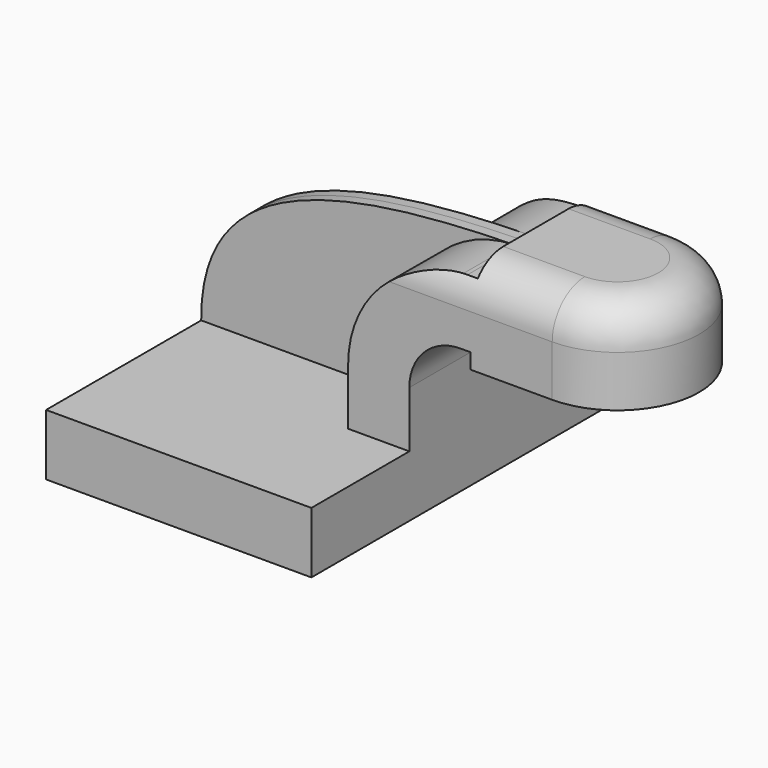
from build123d import *

# Parameters (mm, degrees)
F1_DEPTH = 63.5
F0_W     = 25.4
F0_H     = 19.05
F0_H_2   = 4.7498
F0_H_3   = 4.7752
F2_DEPTH = 25.4
F4_DEPTH = 3.175
F5_R     = 12.7


with BuildPart() as f1:
    # F0 (on Front) → F1 (new body, symmetric)
    with BuildSketch(Plane.XZ):
        Polygon((41.275, -9.525), (41.275, 9.525), (22.225, 9.525), (-41.275, 9.525), (-41.275, -9.525), align=None)
    extrude(amount=F1_DEPTH, both=True)

    # F0 (on Front) → F2 (join, symmetric)
    with BuildSketch(Plane.XZ):
        with BuildLine():
            Line((22.225, 9.525), (41.275, 9.525))
            Line((41.275, 9.525), (41.275, 27.0002))
            ThreePointArc((41.275, 27.0002), (45.9246798487, 38.2255201513), (57.15, 42.8752))
            Line((57.15, 42.8752), (60.325, 42.8752))
            Line((60.325, 42.8752), (60.325, 61.9252))
            Line((60.325, 61.9252), (57.15, 61.9252))
            add(Edge.make_bspline(
                [(55.8906627655, 61.9024878151), (56.3095920905, 61.9105285601), (56.7293746708, 61.9180961221), (57.15, 61.9252)],
                knots=[110.683860184, 110.683860184, 110.683860184, 110.683860184, 111.5045361635, 111.5045361635, 111.5045361635, 111.5045361635], degree=3))
            ThreePointArc((55.8906627655, 61.9024878151), (32.0129956248, 51.2465736679), (22.225, 27.0002))
            Line((22.225, 27.0002), (22.225, 9.525))
        make_face()
        with Locations((73.025, 52.4002)):
            Rectangle(F0_W, F0_H)
        with Locations((73.025, 64.3001)):
            Rectangle(F0_W, F0_H_2)
        with Locations((73.025, 40.4876)):
            Rectangle(F0_W, F0_H_3)
    extrude(amount=F2_DEPTH, both=True)

    # F0 (on Front) → F3 (revolve)
    with BuildSketch(Plane.XZ):
        Polygon((85.725, 61.9252), (85.725, 42.8752), (85.725, 38.1), (111.125, 38.1), (111.125, 66.675), (85.725, 66.675), align=None)
    revolve(axis=Axis((85.725, 0, 52.3875), (0, 0, 1)))

    # F0 (on Front) → F4 (join, symmetric)
    with BuildSketch(Plane.XZ):
        with BuildLine():
            Line((-41.275, 9.525), (22.225, 9.525))
            Line((22.225, 9.525), (22.225, 27.0002))
            ThreePointArc((22.225, 27.0002), (32.0129956248, 51.2465736679), (55.8906627655, 61.9024878151))
            add(Edge.make_bspline(
                [(-41.275, 9.525), (-41.5901642884, 51.126542611), (-0.6099732885, 60.8180394914), (55.8906627655, 61.9024878151)],
                knots=[0, 0, 0, 0, 110.683860184, 110.683860184, 110.683860184, 110.683860184], degree=3))
        make_face()
    extrude(amount=F4_DEPTH, both=True)

    # F5
    f5_edges = [f1.edges().sort_by_distance(p)[0] for p in [
        (85.725, 25.4, 52.3875),
        (73.025, 25.4, 66.675),
        (73.025, -25.4, 66.675),
        (111.125, 0, 66.675),
    ]]
    fillet(f5_edges, radius=F5_R)


solid = f1.part
